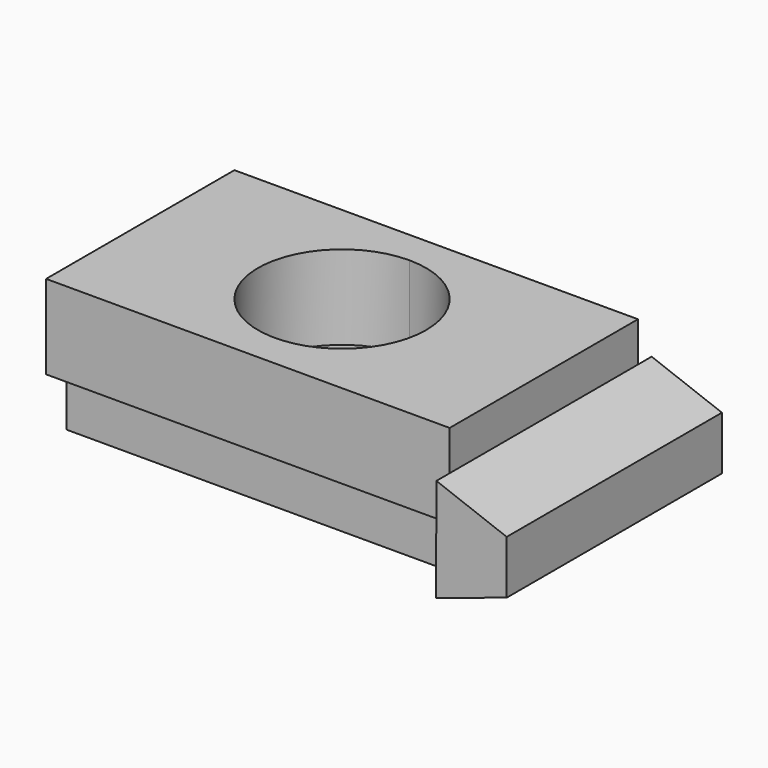
from build123d import *

# Parameters (mm, degrees)
F1_DEPTH = 50
F2_W     = 240
F2_H     = 110
F2_R     = 50
F3_DEPTH = 35
F5_DEPTH = 80


with BuildPart() as f1:
    # F0 (on Top) → F1 (new body)
    with BuildSketch(Plane.XY):
        Polygon((120, 70), (0, 70), (-120, 70), (-120, -70), (120, -70), align=None)
        with BuildLine():
            ThreePointArc((0, 50), (35.3553390593, 35.3553390593), (50, 0))
            ThreePointArc((50, 0), (-35.3553390593, -35.3553390593), (0, 50))
        make_face(mode=Mode.SUBTRACT)
    extrude(amount=-F1_DEPTH)

    # F2 (on face) → F3 (join)
    with BuildSketch(Plane(origin=(0, 0, -50), x_dir=(1, 0, 0), z_dir=(0, 0, -1))):
        Rectangle(F2_W, F2_H)
        Circle(F2_R, mode=Mode.SUBTRACT)
        Circle(F2_R)
    extrude(amount=F3_DEPTH)

    # F4 (on Front) → F5 (join, symmetric)
    with BuildSketch(Plane.XZ):
        Polygon((161.9289219379, -39.3364913762), (120.1279684901, -23.6113723367), (119.9289113283, -84.9194303155), (161.9289219379, -71.184836328), align=None)
    extrude(amount=F5_DEPTH, both=True)


solid = f1.part
